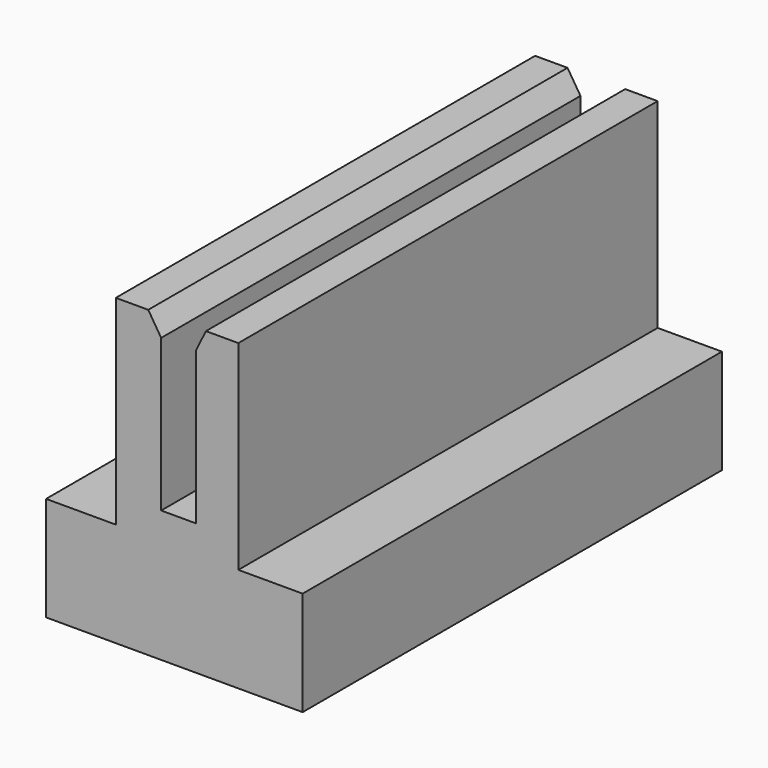
from build123d import *

# Parameters (mm, degrees)
F1_DEPTH = 40.005


# Not quite as in the source:
# - the program builds the solid bodies; features that only make, move or delete a surface that nothing else refers to are left out


with BuildPart() as f1:
    # F0 (on Front) → F1 (new body)
    with BuildSketch(Plane.XZ):
        Polygon((-10.5928385672, 7.9657547176), (-10.5928385672, 0), (8.9905614328, 0), (8.9905614328, 7.9657547176), (4.0834043175, 7.9657547176), (4.0834043175, 23.2057547176), (1.6075200401, 23.2057547176), (0.8385349647, 21.6401405632), (0.8385349647, 10.0401053205), (-1.8070872175, 10.0401053205), (-1.8070872175, 21.6401405632), (-2.7943993919, 23.2057547176), (-5.2702836692, 23.2057547176), (-5.2702836692, 7.9657547176), align=None)
    extrude(amount=F1_DEPTH)


solid = f1.part
